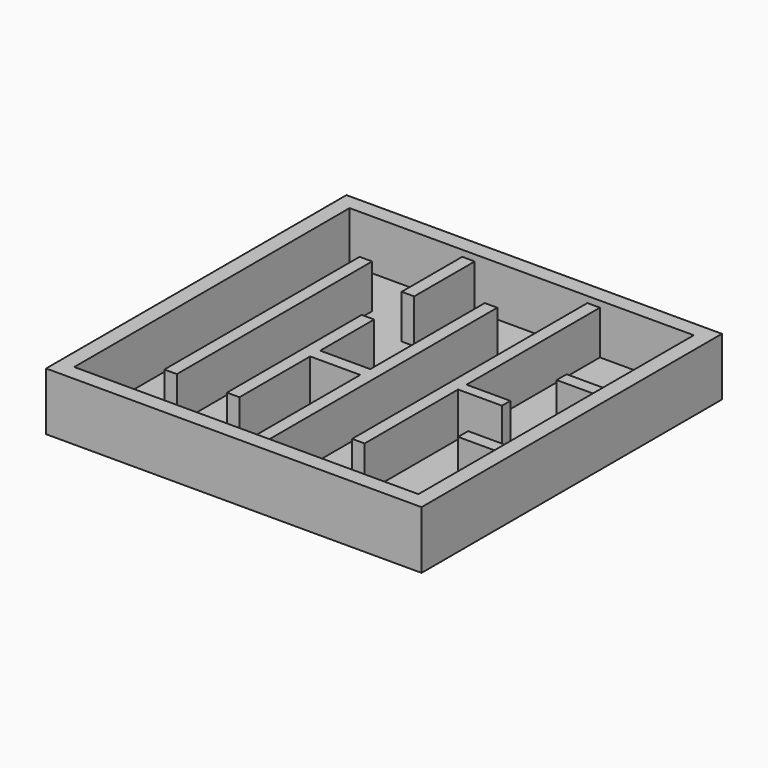
from build123d import *

# Parameters (mm, degrees)
F0_W         = 38.1
F0_H         = 38.1
F1_DEPTH     = 0.79375
F2_W         = 38.1
F2_H         = 38.1
F2_W_2       = 34.925
F2_H_2       = 34.925
F3_DEPTH     = 5.08
F4_W         = 1.27
F4_H         = 24.765
F4_H_2       = 7.0556558254
F4_H_3       = 0.6237175866
F4_W_2       = 5.08
F4_H_4       = 1.27
F4_W_3       = 4.445
F4_H_5       = 1.065895427
F5_DEPTH     = 4.445
F6_TEXT_SIZE = 7.7206124034
F7_DEPTH     = 0.1984375
F8_R         = 1.27
F9_DEPTH     = 0.1984375
F10_R        = 1.27
F11_DEPTH    = 0.1984375


# Not quite as in the source:
# - Text() gives the source's letters only with a copy of the font that has no kerning and outlines rounded to 1/6400 em; it was checked with that copy


with BuildPart() as f1:
    # F0 (on Top) → F1 (new body)
    with BuildSketch(Plane.XY):
        with Locations((0, -5.6688048375)):
            Rectangle(F0_W, F0_H)
    extrude(amount=F1_DEPTH)

    # F2 (on face) → F3 (join)
    with BuildSketch(Plane.XY.offset(0.79375)):
        with Locations((0, -5.6688048375)):
            Rectangle(F2_W, F2_H)
        with Locations((0, -5.6688048375)):
            Rectangle(F2_W_2, F2_H_2, mode=Mode.SUBTRACT)
    extrude(amount=F3_DEPTH)

    # F4 (on face) → F5 (join)
    with BuildSketch(Plane.XY.offset(0.79375)):
        with Locations((-11.7475, -5.6688048375)):
            Rectangle(F4_W, F4_H)
        Polygon((-4.7625, -18.0513048375), (-4.7625, -9.0778646991), (-4.7625, -7.8078646991), (-4.7625, -0.9656782495), (-6.0325, -0.9656782495), (-6.0325, -18.0513048375), align=None)
        with Locations((-5.3975, 8.2658672498)):
            Rectangle(F4_W, F4_H_2)
        with Locations((-5.3975, 4.4261805438)):
            Rectangle(F4_W, F4_H_3)
        Polygon((0.3175, -9.0778646991), (0.3175, -23.1313048375), (1.5875, -23.1313048375), (1.5875, 6.7136951625), (0.3175, 6.7136951625), (0.3175, -7.8078646991), align=None)
        with Locations((-2.2225, -8.4428646991)):
            Rectangle(F4_W_2, F4_H_4)
        Polygon((7.9375, 11.7936951625), (6.6675, 11.7936951625), (6.6675, -18.0513048375), (7.9375, -18.0513048375), (7.9375, -6.1905221082), (7.9375, -5.1246266812), align=None)
        with Locations((10.16, -5.6575743947)):
            Rectangle(F4_W_3, F4_H_5)
        with Locations((15.24, 0.5903733188)):
            Rectangle(F4_W_3, F4_H_4)
        with Locations((15.24, -11.9055221082)):
            Rectangle(F4_W_3, F4_H_4)
    extrude(amount=F5_DEPTH)

    # F6 (on face) → F7 (cut, symmetric)
    with BuildSketch(Plane(origin=(0, 0, 0), x_dir=(1, 0, 0), z_dir=(0, 0, -1))):
        with Locations((-10.6710875407, 1.9517951878)):
            Text('David', F6_TEXT_SIZE, font='Open Sans', font_style=FontStyle.BOLD, text_align=(TextAlign.LEFT, TextAlign.BOTTOM))
    extrude(amount=F7_DEPTH, both=True, mode=Mode.SUBTRACT)

    # F8 (on face) → F9 (cut, symmetric)
    with BuildSketch(Plane.XY.offset(0.79375)):
        with Locations((-14.9225, -20.3798897564)):
            Circle(F8_R)
    extrude(amount=F9_DEPTH, both=True, mode=Mode.SUBTRACT)

    # F10 (on face) → F11 (cut, symmetric)
    with BuildSketch(Plane.XY.offset(0.79375)):
        with Locations((12.7, 6.8013439886)):
            Circle(F10_R)
    extrude(amount=F11_DEPTH, both=True, mode=Mode.SUBTRACT)


solid = f1.part
